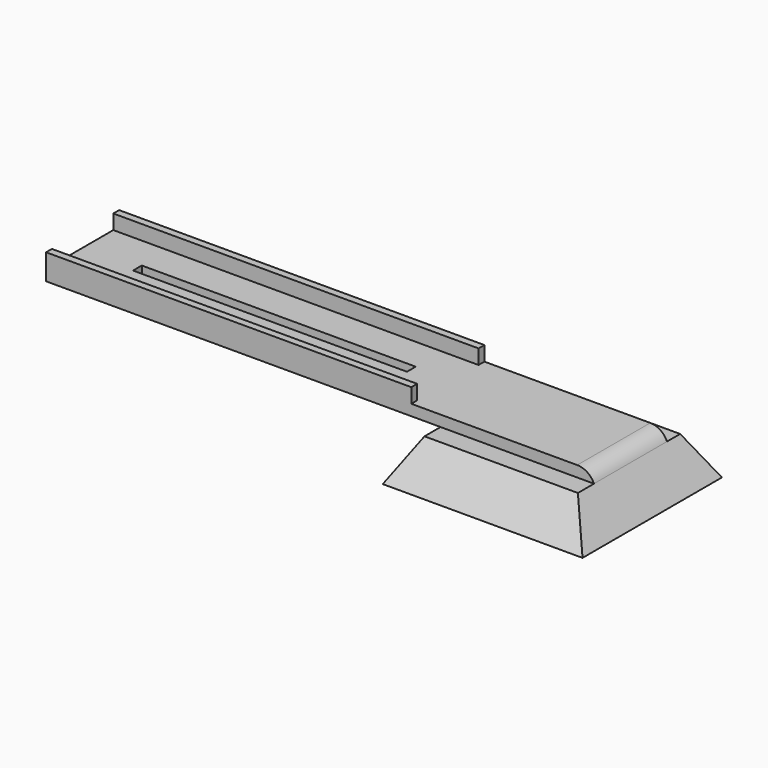
from build123d import *

# Parameters (mm, degrees)
F0_W        = 150
F0_H        = 25
F1_DEPTH    = 3
F2_W        = 100
F2_H        = 2
F3_DEPTH    = 7
F4_W        = 42
F4_H        = 5.5
F4_H_2      = 29.5
F5_DEPTH    = 11
F5_TAPER    = -30
F6_W        = 75
F6_H        = 3
F7_DEPTH    = 7.001
F8_T1_DEPTH = 47.9128784748


# Not quite as in the source:
# - a fillet or chamfer that OpenCascade refuses, or shapes differently, is made with other operations: its cross-section is extruded or revolved along the edge and cut away or added


with BuildPart() as f1:
    # F0 (on Top) → F1 (new body)
    with BuildSketch(Plane.XY):
        with Locations((75, 12.5)):
            Rectangle(F0_W, F0_H)
    extrude(amount=F1_DEPTH)

    # F2 (on Top) → F3 (join)
    with BuildSketch(Plane.XY):
        with Locations((50, 24)):
            Rectangle(F2_W, F2_H)
        with Locations((50, 1)):
            Rectangle(F2_W, F2_H)
    extrude(amount=F3_DEPTH)

    # F4 (on Top) → F5 (join)
    with BuildSketch(Plane.XY):
        with Locations((129, -2.75)):
            Rectangle(F4_W, F4_H)
        with Locations((129, 14.75)):
            Rectangle(F4_W, F4_H_2)
    extrude(amount=-F5_DEPTH, taper=F5_TAPER)

    # F6 (on Top) → F7 (cut, through all)
    with BuildSketch(Plane.XY):
        with Locations((52.5, 12.5)):
            Rectangle(F6_W, F6_H)
    extrude(amount=F7_DEPTH, mode=Mode.SUBTRACT)

    # F8: fillet of radius 5 on 1 edges, made by hand

    # F8_s2 → F8_t1 (cut)
    with BuildSketch(Plane.XZ.offset(-36.4564392374)):
        with BuildLine():
            ThreePointArc((145.417424305, 3), (148.1560370926, 2.1833001327), (150, 0))
            Line((150, 0), (150.0916515139, 0.04))
            ThreePointArc((150.0916515139, 0.04), (150.1, 1.5), (150.1, 3))
            Line((150.1, 3), (150, 3.1))
            Line((150, 3.1), (145.417424305, 3.1))
            Line((145.417424305, 3.1), (145.417424305, 3))
        make_face()
    extrude(amount=F8_T1_DEPTH, mode=Mode.SUBTRACT)


solid = f1.part
